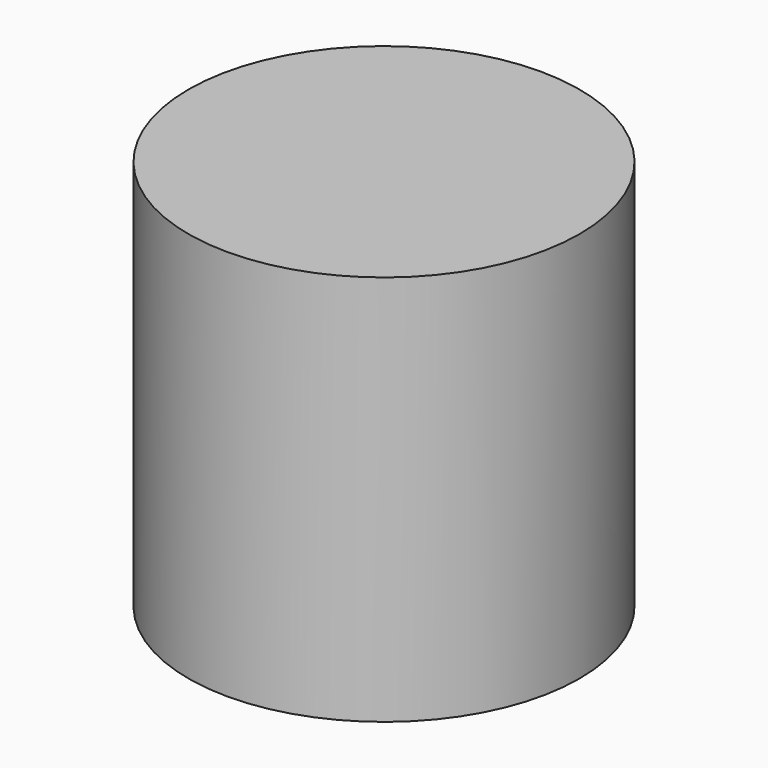
from build123d import *

# Parameters (mm, degrees)
F0_R     = 12.7
F1_DEPTH = 25.4


# Not quite as in the source:
# - the program builds the solid bodies; features that only make, move or delete a surface that nothing else refers to are left out


with BuildPart() as f1:
    # F0 (on Top) → F1 (new body)
    with BuildSketch(Plane.XY):
        Circle(F0_R)
    extrude(amount=-F1_DEPTH)


solid = f1.part
